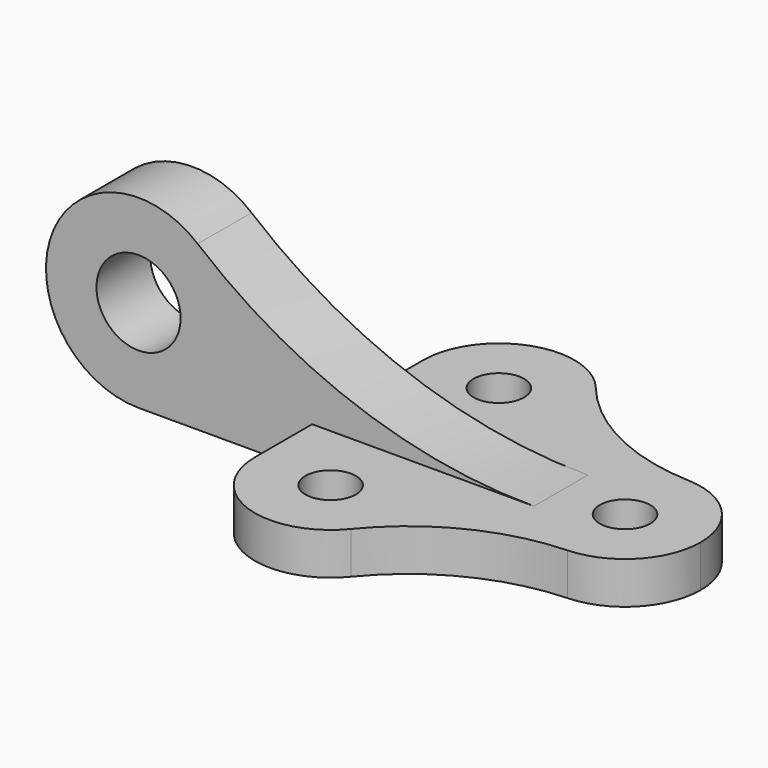
from build123d import *

# Parameters (mm, degrees)
F0_R     = 6
F1_DEPTH = 10
F2_R     = 10
F3_DEPTH = 8


# Not quite as in the source:
# - after a boolean that leaves OpenCascade's solid faulty, fix() repairs it
# - ends of sketch curves that miss each other by under 0.0002 mm in the source are joined


with BuildPart() as f1:
    # F0 (on Top) → F1 (new body)
    with BuildSketch(Plane.XY):
        with BuildLine():
            ThreePointArc((-67.9963028434, 24.6351932456), (-49.8175872558, 7.0009243129), (-32, 25))
            ThreePointArc((-32, 25), (-33.0411037726, 31.0328963813), (-36.0439820831, 36.3679181868))
            ThreePointArc((-36.0439820831, 36.3679181868), (-55.8594566993, 42.0195995014), (-67.9962482966, 25.3674877532))
            Line((-67.9962482966, 25.3674877532), (-67.9963028434, 24.6351932456))
        make_face()
        with Locations((-50, 25)):
            Circle(F0_R, mode=Mode.SUBTRACT)
        with BuildLine():
            ThreePointArc((-36.0439820831, 36.3679181868), (-33.0411037726, 31.0328963813), (-32, 25))
            ThreePointArc((-32, 25), (-49.8175872558, 7.0009243129), (-67.9963028434, 24.6351932456))
            Line((-67.9963028434, 24.6351932456), (-67.9999999501, -24.9986592232))
            ThreePointArc((-67.9999999501, -24.9986592232), (-49.9993296116, -7.0000000125), (-32, -25))
            ThreePointArc((-32, -25), (-33.0411037726, -31.0328963813), (-36.0439820831, -36.3679181868))
            ThreePointArc((-36.0439820831, -36.3679181868), (-19.6379454221, -23.2241091558), (0.7207237993, -17.9855652456))
            ThreePointArc((0.7207237993, -17.9855652456), (-18, 0), (0.7207237993, 17.9855652456))
            ThreePointArc((0.7207237993, 17.9855652456), (-19.6379454221, 23.2241091558), (-36.0439820831, 36.3679181868))
        make_face()
        with BuildLine():
            ThreePointArc((-67.9962482966, 25.3674877532), (-67.9999999501, 25.0013407768), (-67.9963028434, 24.6351932456))
            Line((-67.9963028434, 24.6351932456), (-67.9962482966, 25.3674877532))
        make_face()
        with BuildLine():
            ThreePointArc((18, 0), (12.9802355215, 12.4705046332), (0.7207237993, 17.9855652456))
            ThreePointArc((0.7207237993, 17.9855652456), (-18, 0), (0.7207237993, -17.9855652456))
            ThreePointArc((0.7207237993, -17.9855652456), (12.9802355215, -12.4705046332), (18, 0))
        make_face()
        Circle(F0_R, mode=Mode.SUBTRACT)
        with BuildLine():
            ThreePointArc((-32, -25), (-49.9993296116, -7.0000000125), (-67.9999999501, -24.9986592232))
            ThreePointArc((-67.9999999501, -24.9986592232), (-56.0335279909, -41.9586715277), (-36.0439820831, -36.3679181868))
            ThreePointArc((-36.0439820831, -36.3679181868), (-33.0411037726, -31.0328963813), (-32, -25))
        make_face()
        with Locations((-50, -25)):
            Circle(F0_R, mode=Mode.SUBTRACT)
    extrude(amount=F1_DEPTH)

    # F2 (on Front) → F3 (join, symmetric)
    with BuildSketch(Plane.XZ):
        with BuildLine():
            ThreePointArc((-15.2580020124, 10), (-57.7665045632, 17.4498948921), (-95.2080650977, 38.9115646259))
            ThreePointArc((-95.2080650977, 38.9115646259), (-129.9613786248, 29.5000426212), (-109.3187257013, 3.53696e-05))
            Line((-109.3187257013, 3.53696e-05), (-15.2580020124, 0))
            Line((-15.2580020124, 0), (-15.2580020124, 10))
        make_face()
        with Locations((-109.2792762007, 22)):
            Circle(F2_R, mode=Mode.SUBTRACT)
        with BuildLine():
            ThreePointArc((-109.3187257013, 3.53696e-05), (-93.7368807774, 6.4297095561), (-87.2792762007, 22))
            ThreePointArc((-87.2792762007, 22), (-89.3598554729, 31.3389869829), (-95.2080650977, 38.9115646259))
            ThreePointArc((-95.2080650977, 38.9115646259), (-57.7665045632, 17.4498948921), (-15.2580020124, 10))
            Line((-15.2580020124, 10), (-15.2580020124, 0))
            Line((-15.2580020124, 0), (-109.3187257013, 3.53696e-05))
        make_face(mode=Mode.SUBTRACT)
    extrude(amount=F3_DEPTH, both=True)

    add(f1.part.fix(), mode=Mode.REPLACE)


solid = f1.part
